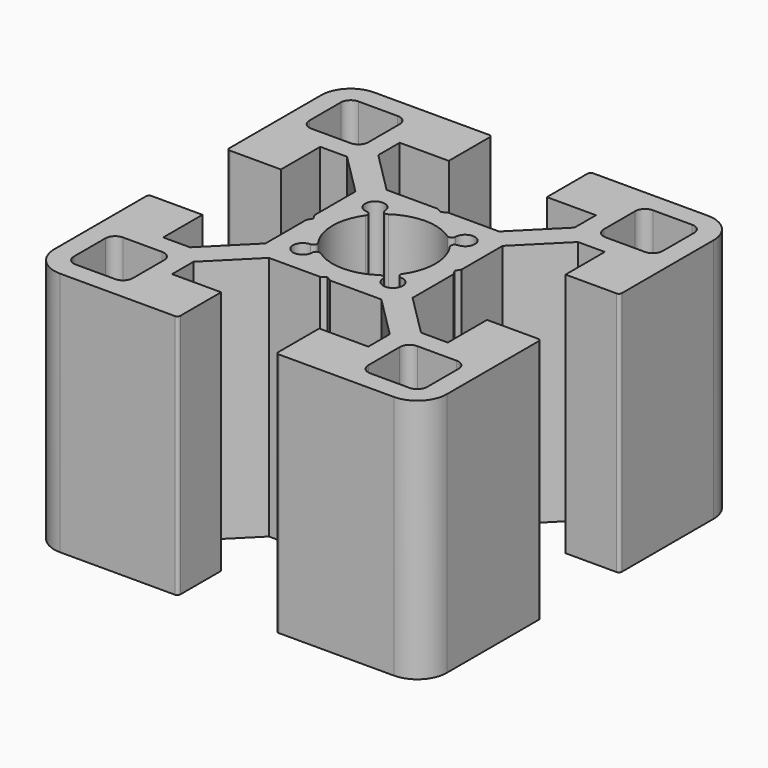
from build123d import *

# Parameters (mm, degrees)
F1_DEPTH = 25


# Not quite as in the source:
# - ends of sketch curves that miss each other by under 0.0002 mm in the source are joined


with BuildPart() as f1:
    # F0 (on Top) → F1 (new body)
    with BuildSketch(Plane.XY):
        with BuildLine():
            Line((-18.380952, 17.5), (-13.180955, 17.5))
            ThreePointArc((-13.180955, 17.5), (-12.9688229656, 17.5878709656), (-12.880955, 17.800003))
            Line((-12.880955, 17.800003), (-12.880952, 29.500001))
            ThreePointArc((-12.880952, 29.500001), (-13.7596316564, 31.6213203436), (-15.880952, 32.5))
            Line((-15.880952, 32.5), (-27.580952, 32.5))
            ThreePointArc((-27.580952, 32.5), (-27.7930840344, 32.4121320344), (-27.880952, 32.2))
            Line((-27.880952, 32.2), (-27.880952, 27))
            Line((-27.880952, 27), (-22.880952, 27))
            Line((-22.880952, 27), (-22.880952, 24.267777))
            Line((-22.880952, 24.267777), (-27.148715, 20))
            Line((-27.148715, 20), (-32.361337, 20))
            Line((-32.361337, 20), (-32.880952, 19.7))
            Line((-32.880952, 19.7), (-33.400567, 20))
            Line((-33.400567, 20), (-38.613181, 20))
            Line((-38.613181, 20), (-42.880937, 24.267771))
            Line((-42.880937, 24.267771), (-42.880952, 27))
            Line((-42.880952, 27), (-37.880952, 27))
            Line((-37.880952, 27), (-37.880952, 32.2))
            ThreePointArc((-37.880952, 32.2), (-37.9688199656, 32.4121320344), (-38.180952, 32.5))
            Line((-38.180952, 32.5), (-49.880952, 32.5))
            ThreePointArc((-49.880952, 32.5), (-52.0022723436, 31.6213203436), (-52.880952, 29.5))
            Line((-52.880952, 29.5), (-52.880952, 17.800003))
            ThreePointArc((-52.880952, 17.800003), (-52.7930810344, 17.5878709656), (-52.580949, 17.500003))
            Line((-52.580949, 17.500003), (-47.380937, 17.5))
            Line((-47.380937, 17.5), (-47.380952, 22.5))
            Line((-47.380952, 22.5), (-44.648728, 22.500001))
            Line((-44.648728, 22.500001), (-40.380952, 18.232248))
            Line((-40.380952, 18.232248), (-40.380952, 13.019615))
            Line((-40.380952, 13.019615), (-40.080952, 12.5))
            Line((-40.080952, 12.5), (-40.380952, 11.980385))
            Line((-40.380952, 11.980385), (-40.380952, 6.767753))
            Line((-40.380952, 6.767753), (-44.648721, 2.499994))
            Line((-44.648721, 2.499994), (-47.380937, 2.500006))
            Line((-47.380937, 2.500006), (-47.380952, 7.5))
            Line((-47.380952, 7.5), (-52.580949, 7.5))
            ThreePointArc((-52.580949, 7.5), (-52.7930810344, 7.4121290344), (-52.880949, 7.199997))
            Line((-52.880949, 7.199997), (-52.880952, -4.5))
            ThreePointArc((-52.880952, -4.5), (-52.0022723436, -6.6213203436), (-49.880952, -7.5))
            Line((-49.880952, -7.5), (-38.180955, -7.5))
            ThreePointArc((-38.180955, -7.5), (-37.9688199656, -7.4121320344), (-37.880952, -7.2))
            Line((-37.880952, -7.2), (-37.880952, -2))
            Line((-37.880952, -2), (-42.880952, -2))
            Line((-42.880952, -2), (-42.880952, 0.732224))
            Line((-42.880952, 0.732224), (-38.613182, 5))
            Line((-38.613182, 5), (-33.400567, 5))
            Line((-33.400567, 5), (-32.880952, 5.3))
            Line((-32.880952, 5.3), (-32.361337, 5))
            Line((-32.361337, 5), (-27.148714, 5))
            Line((-27.148714, 5), (-22.880944, 0.732225))
            Line((-22.880944, 0.732225), (-22.880952, -2))
            Line((-22.880952, -2), (-27.880952, -2))
            Line((-27.880952, -2), (-27.880952, -7.2))
            ThreePointArc((-27.880952, -7.2), (-27.7930840344, -7.4121320344), (-27.580952, -7.5))
            Line((-27.580952, -7.5), (-15.880952, -7.5))
            ThreePointArc((-15.880952, -7.5), (-13.7596316564, -6.6213203436), (-12.880952, -4.5))
            Line((-12.880952, -4.5), (-12.880952, 7.199997))
            ThreePointArc((-12.880952, 7.199997), (-12.9688229656, 7.4121290344), (-13.180955, 7.499997))
            Line((-13.180955, 7.499997), (-18.380952, 7.5))
            Line((-18.380952, 7.5), (-18.380952, 2.5))
            Line((-18.380952, 2.5), (-21.113175, 2.499999))
            Line((-21.113175, 2.499999), (-25.380952, 6.76777))
            Line((-25.380952, 6.76777), (-25.380952, 11.980385))
            Line((-25.380952, 11.980385), (-25.680952, 12.5))
            Line((-25.680952, 12.5), (-25.380952, 13.019615))
            Line((-25.380952, 13.019615), (-25.380952, 18.232231))
            Line((-25.380952, 18.232231), (-21.113175, 22.5))
            Line((-21.113175, 22.5), (-18.380952, 22.5))
            Line((-18.380952, 22.5), (-18.380952, 17.5))
        make_face()
        with BuildLine():
            ThreePointArc((-50.880952, -0.5), (-50.5880587812, 0.2071067812), (-49.880952, 0.5))
            Line((-49.880952, 0.5), (-45.880937, 0.5))
            ThreePointArc((-45.880937, 0.5), (-45.1738452188, 0.2071007812), (-44.880952, -0.500006))
            Line((-44.880952, -0.500006), (-44.880952, -4.5))
            ThreePointArc((-44.880952, -4.5), (-45.1738452188, -5.2071067812), (-45.880952, -5.5))
            Line((-45.880952, -5.5), (-49.880952, -5.5))
            ThreePointArc((-49.880952, -5.5), (-50.5880587812, -5.2071067812), (-50.880952, -4.5))
            Line((-50.880952, -4.5), (-50.880952, -0.5))
        make_face(mode=Mode.SUBTRACT)
        with BuildLine():
            Line((-14.880952, -0.499999), (-14.880952, -4.5))
            ThreePointArc((-14.880952, -4.5), (-15.1738452188, -5.2071067812), (-15.880952, -5.5))
            Line((-15.880952, -5.5), (-19.880952, -5.5))
            ThreePointArc((-19.880952, -5.5), (-20.5880587812, -5.2071067812), (-20.880952, -4.5))
            Line((-20.880952, -4.5), (-20.880952, -0.499999))
            ThreePointArc((-20.880952, -0.499999), (-20.5880587812, 0.2071077812), (-19.880952, 0.500001))
            Line((-19.880952, 0.500001), (-15.880952, 0.500001))
            ThreePointArc((-15.880952, 0.500001), (-15.1738452188, 0.2071077812), (-14.880952, -0.499999))
        make_face(mode=Mode.SUBTRACT)
        with BuildLine():
            ThreePointArc((-37.1869759587, 9.4965590288), (-38.130952, 12.5000067994), (-37.186968179, 15.5034521248))
            ThreePointArc((-37.186968179, 15.5034521248), (-37.1632332946, 15.8875474988), (-37.4865620002, 16.0962359962))
            ThreePointArc((-37.4865620002, 16.0962359962), (-38.1843329758, 17.8032195777), (-36.4771934562, 17.1058309956))
            ThreePointArc((-36.4771934562, 17.1058309956), (-36.2684563797, 16.7822649872), (-35.8841472989, 16.8061954442))
            ThreePointArc((-35.8841472989, 16.8061954442), (-32.8808765483, 17.7499999995), (-29.8776329856, 16.8061090207))
            ThreePointArc((-29.8776329856, 16.8061090207), (-29.4930868042, 16.7824504958), (-29.2847080657, 17.1065090027))
            ThreePointArc((-29.2847080657, 17.1065090027), (-27.578165673, 17.8038098657), (-28.2729980022, 16.0962611865))
            ThreePointArc((-28.2729980022, 16.0962611865), (-28.5981729586, 15.8885199872), (-28.5748681009, 15.5033549322))
            ThreePointArc((-28.5748681009, 15.5033549322), (-27.6309520001, 12.5000377259), (-28.5748248894, 9.4967069229))
            ThreePointArc((-28.5748248894, 9.4967069229), (-28.5986102211, 9.1123426938), (-28.2748899919, 8.9037591925))
            ThreePointArc((-28.2748899919, 8.9037591925), (-27.577743326, 7.1966121229), (-29.2847147364, 7.8941890025))
            ThreePointArc((-29.2847147364, 7.8941890025), (-29.493086142, 8.2175661088), (-29.8770772102, 8.1942793139))
            ThreePointArc((-29.8770772102, 8.1942793139), (-32.8797784079, 7.2500001312), (-35.8829017766, 8.1929363205))
            ThreePointArc((-35.8829017766, 8.1929363205), (-36.2677680781, 8.2180997059), (-36.4771928672, 7.8942229943))
            ThreePointArc((-36.4771928672, 7.8942229943), (-38.1841540665, 7.1966015182), (-37.4870140032, 8.9037593199))
            ThreePointArc((-37.4870140032, 8.9037593199), (-37.1633341924, 9.1122631312), (-37.1869759587, 9.4965590288))
        make_face(mode=Mode.SUBTRACT)
        with BuildLine():
            Line((-49.880952, 30.5), (-45.880952, 30.5))
            ThreePointArc((-45.880952, 30.5), (-45.1738452188, 30.2071067812), (-44.880952, 29.5))
            Line((-44.880952, 29.5), (-44.880952, 25.5))
            ThreePointArc((-44.880952, 25.5), (-45.1738452188, 24.7928932188), (-45.880952, 24.5))
            Line((-45.880952, 24.5), (-49.880952, 24.5))
            ThreePointArc((-49.880952, 24.5), (-50.5880587812, 24.7928932188), (-50.880952, 25.5))
            Line((-50.880952, 25.5), (-50.880952, 29.5))
            ThreePointArc((-50.880952, 29.5), (-50.5880587812, 30.2071067812), (-49.880952, 30.5))
        make_face(mode=Mode.SUBTRACT)
        with BuildLine():
            ThreePointArc((-15.880952, 30.5), (-15.1738452188, 30.2071067812), (-14.880952, 29.5))
            Line((-14.880952, 29.5), (-14.880952, 25.5))
            ThreePointArc((-14.880952, 25.5), (-15.1738452188, 24.7928932188), (-15.880952, 24.5))
            Line((-15.880952, 24.5), (-19.880967, 24.5))
            ThreePointArc((-19.880967, 24.5), (-20.5880587812, 24.7928892188), (-20.880952, 25.499996))
            Line((-20.880952, 25.499996), (-20.880952, 29.5))
            ThreePointArc((-20.880952, 29.5), (-20.5880587812, 30.2071067812), (-19.880952, 30.5))
            Line((-19.880952, 30.5), (-15.880952, 30.5))
        make_face(mode=Mode.SUBTRACT)
    extrude(amount=F1_DEPTH)


solid = f1.part
